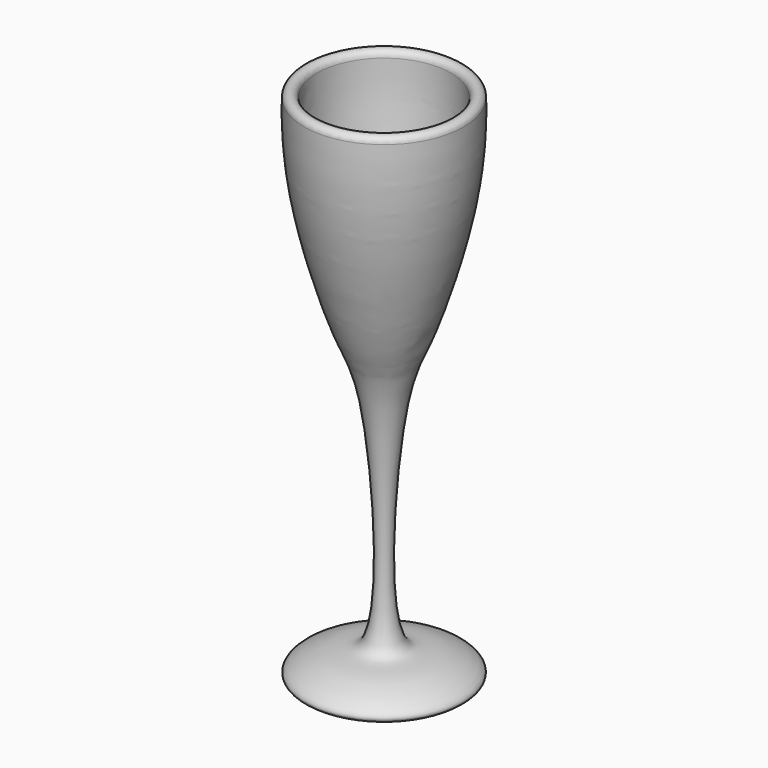
from build123d import *

# Parameters (mm, degrees)
F3_R = 1.27


# Not quite as in the source:
# - a fillet or chamfer that OpenCascade refuses, or shapes differently, is made with other operations: its cross-section is extruded or revolved along the edge and cut away or added


with BuildPart() as f1:
    # F0 (on Front) → F1 (revolve)
    with BuildSketch(Plane.XZ):
        with BuildLine():
            add(Edge.make_bspline(
                [(-8.9504094794, 65.7735615969), (-10.1002320619, 60.8536000039), (-12.4755391669, 50.6899278797), (-13.8751598665, 32.4029277885), (-11.7808838385, 16.0086835126), (-7.7777227562, -8.5297782559), (-1.9542906374, -7.6339367652), (0, -7.3333005421)],
                knots=[0, 0, 0, 0, 0.2021725958, 0.4176487838, 0.6390547122, 0.8788700577, 1, 1, 1, 1], degree=3))
            Line((-8.9504094794, 65.7735615969), (-10.9729282558, 65.7735615969))
            add(Edge.make_bspline(
                [(-10.9729282558, 65.7735615969), (-12.099165275, 61.3250150964), (-14.5014764715, 51.8360772581), (-16.49137647, 33.1978948569), (-14.807091019, 14.6435085166), (-7.7382118319, -8.3275453358), (-2.5497359939, -16.585006741), (0.2857630852, -63.3983935632), (-8.2838276602, -61.0955024284), (-21.4551680801, -67.269553999), (-7.9365971981, -68.3336521274), (0, -68.9583718777)],
                knots=[0, 0, 0, 0, 0.1037083822, 0.2212143656, 0.3430815454, 0.4721008542, 0.5697545725, 0.7454098678, 0.8122406833, 0.8897686686, 1, 1, 1, 1], degree=3))
            Line((0, -68.9583718777), (0, -7.3333005421))
        make_face()
    revolve(axis=Axis((0, 0, -1.5924051404), (0, 0, -1)))

    # F2: fillet of radius 5.08 on 1 edges, made by hand

    # F2_s1 → F2_t2 (revolve, cut)
    with BuildSketch(Plane.XZ):
        with BuildLine():
            ThreePointArc((-11.8344780682, 62.3448166475), (-10.7908673283, 64.3943207448), (-8.9504094794, 65.7735615969))
            Line((-8.9504094794, 65.7735615969), (-8.9913521089, 65.8665468704))
            ThreePointArc((-8.9913521089, 65.8665468704), (-9.9616688676, 65.8751615969), (-10.9729282558, 65.8751615969))
            Line((-10.9729282558, 65.8751615969), (-11.0714208398, 65.7984969312))
            ThreePointArc((-11.0714208398, 65.7984969312), (-11.5045182242, 64.0845684134), (-11.9331020694, 62.3692270221))
            Line((-11.9331020694, 62.3692270221), (-11.8344780682, 62.3448166475))
        make_face()
    revolve(axis=Axis((0, 0, 65.7735615969), (0, 0, -1)), mode=Mode.SUBTRACT)

    # F3
    f3_edges = [f1.edges().sort_by_distance(p)[0] for p in [
        (8.950409, 0, 65.773562),
    ]]
    fillet(f3_edges, radius=F3_R)


solid = f1.part
